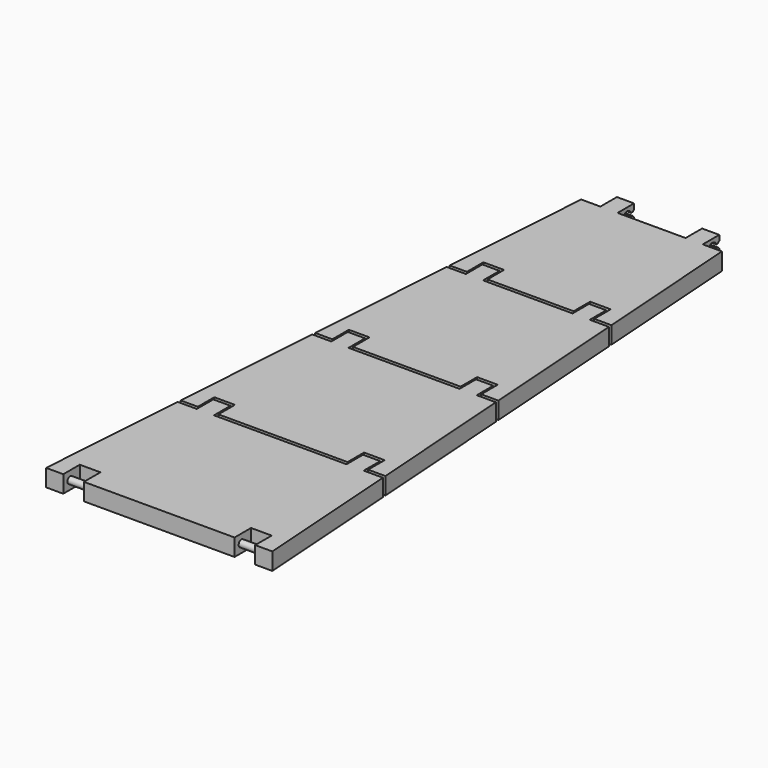
from build123d import *

# Parameters (mm, degrees)
F1_DEPTH  = 5
F12_START = -5.7
F10_R     = 1
F12_DEPTH = 62
F13_START = -5.5
F9_R      = 1.5
F9_R_2    = 1
F13_DEPTH = 55.3
F14_START = -6
F14_DEPTH = 56.6
F15_START = -6.3
F8_R      = 1.5
F8_R_2    = 1
F15_DEPTH = 49.5
F16_START = -5.7
F16_DEPTH = 49
F17_START = -6
F7_R      = 1.5
F7_R_2    = 1
F17_DEPTH = 43.6
F18_START = -5.7
F18_DEPTH = 42.3
F19_DEPTH = 45.5
F20_SIZE  = 0.5


with BuildPart() as f1:
    # F0 (on Top) → F1 (new body)
    with BuildSketch(Plane.XY):
        Polygon((-20.4571957112, 87.1), (-23.5168766766, 43.1), (-18.5168766766, 43.1), (-18.5168766766, 49.1), (-12.5168766766, 49.1), (-12.5168766766, 43.1), (12.5168766766, 43.1), (12.5168766766, 49.1), (18.5168766766, 49.1), (18.5168766766, 43.1), (23.5168766766, 43.1), (20.4571957112, 87.1), (14.8876575074, 87.1), (14.8876575074, 93.1), (9.8876575074, 93.1), (9.8876575074, 87.1), (-9.8876575074, 87.1), (-9.8876575074, 93.1), (-14.8876575074, 93.1), (-14.8876575074, 87.1), align=None)
    extrude(amount=F1_DEPTH)



with BuildPart() as f1b:
    # F0 (on Top) → F1, piece 2 (new body)
    with BuildSketch(Plane.XY):
        Polygon((-23.5864148803, 42.1), (-26.6460958457, -1.9), (-21.6460958457, -1.9), (-21.6460958457, 4.1), (-15.6460958457, 4.1), (-15.6460958457, -1.9), (15.6460958457, -1.9), (15.6460958457, 4.1), (21.6460958457, 4.1), (21.6460958457, -1.9), (26.6460958457, -1.9), (23.5864148803, 42.1), (18.0168766766, 42.1), (18.0168766766, 48.1), (13.0168766766, 48.1), (13.0168766766, 42.1), (-13.0168766766, 42.1), (-13.0168766766, 48.1), (-18.0168766766, 48.1), (-18.0168766766, 42.1), align=None)
    extrude(amount=F1_DEPTH)



with BuildPart() as f1c:
    # F0 (on Top) → F1, piece 3 (new body)
    with BuildSketch(Plane.XY):
        Polygon((-26.7156340495, -2.9), (-29.7753150149, -46.9), (-24.7753150149, -46.9), (-24.7753150149, -40.9), (-18.7753150149, -40.9), (-18.7753150149, -46.9), (18.7753150149, -46.9), (18.7753150149, -40.9), (24.7753150149, -40.9), (24.7753150149, -46.9), (29.7753150149, -46.9), (26.7156340495, -2.9), (21.1460958457, -2.9), (21.1460958457, 3.1), (16.1460958457, 3.1), (16.1460958457, -2.9), (-16.1460958457, -2.9), (-16.1460958457, 3.1), (-21.1460958457, 3.1), (-21.1460958457, -2.9), align=None)
    extrude(amount=F1_DEPTH)



with BuildPart() as f1d:
    # F0 (on Top) → F1, piece 4 (new body)
    with BuildSketch(Plane.XY):
        Polygon((-29.8448532186, -47.9), (-32.904534184, -91.9), (-27.904534184, -91.9), (-27.904534184, -85.9), (-21.904534184, -85.9), (-21.904534184, -91.9), (21.904534184, -91.9), (21.904534184, -85.9), (27.904534184, -85.9), (27.904534184, -91.9), (32.904534184, -91.9), (29.8448532186, -47.9), (24.2753150149, -47.9), (24.2753150149, -41.9), (19.2753150149, -41.9), (19.2753150149, -47.9), (-19.2753150149, -47.9), (-19.2753150149, -41.9), (-24.2753150149, -41.9), (-24.2753150149, -47.9), align=None)
    extrude(amount=F1_DEPTH)

    # F10 (on offset) → F12 (join)
    with BuildSketch(Plane.YZ.offset(36.904534184).offset(F12_START)):
        with Locations((-89.4, 2.5)):
            Circle(F10_R)
    extrude(amount=-F12_DEPTH)

    # F9 (on offset) → F13 (cut)
    with BuildSketch(Plane.YZ.offset(34.2753150149).offset(F13_START)):
        with Locations((-44.4, 2.5)):
            Circle(F9_R)
        with Locations((-44.4, 2.5)):
            Circle(F9_R_2, mode=Mode.SUBTRACT)
    extrude(amount=-F13_DEPTH, mode=Mode.SUBTRACT)


with BuildPart() as f1c_1:
    add(f1c.part)

    add(f1d.part)  # F14 merges F1d
    # F9 (on offset) → F14 (join)
    with BuildSketch(Plane.YZ.offset(34.2753150149).offset(F14_START)):
        with Locations((-44.4, 2.5)):
            Circle(F9_R_2)
    extrude(amount=-F14_DEPTH)

    # F8 (on offset) → F15 (cut)
    with BuildSketch(Plane.YZ.offset(31.1460958457).offset(F15_START)):
        with Locations((0.6, 2.5)):
            Circle(F8_R)
        with Locations((0.6, 2.5)):
            Circle(F8_R_2, mode=Mode.SUBTRACT)
    extrude(amount=-F15_DEPTH, mode=Mode.SUBTRACT)


with BuildPart() as f1b_1:
    add(f1b.part)

    add(f1c_1.part)  # F16 merges F1c
    # F8 (on offset) → F16 (join)
    with BuildSketch(Plane.YZ.offset(31.1460958457).offset(F16_START)):
        with Locations((0.6, 2.5)):
            Circle(F8_R_2)
    extrude(amount=-F16_DEPTH)

    # F7 (on offset) → F17 (cut)
    with BuildSketch(Plane.YZ.offset(28.0168766766).offset(F17_START)):
        with Locations((45.6, 2.5)):
            Circle(F7_R)
        with Locations((45.6, 2.5)):
            Circle(F7_R_2, mode=Mode.SUBTRACT)
    extrude(amount=-F17_DEPTH, mode=Mode.SUBTRACT)


with BuildPart() as f1_1:
    add(f1.part)

    add(f1b_1.part)  # F18 merges F1b
    # F7 (on offset) → F18 (join)
    with BuildSketch(Plane.YZ.offset(28.0168766766).offset(F18_START)):
        with Locations((45.6, 2.5)):
            Circle(F7_R_2)
    extrude(amount=-F18_DEPTH)

    # F11 (on offset) → F19 (cut)
    with BuildSketch(Plane.YZ.offset(24.8876575074)):
        with BuildLine():
            Line((95.6, 3), (92.0142135624, 3))
            ThreePointArc((92.0142135624, 3), (90.4708684127, 3.9944313411), (89.1209800542, 2.75))
            Line((89.1209800542, 2.75), (88.1, 2.75))
            Line((88.1, 2.75), (88.1, 2.25))
            Line((88.1, 2.25), (89.1209800542, 2.25))
            ThreePointArc((89.1209800542, 2.25), (90.4708684127, 1.0055686589), (92.0142135624, 2))
            Line((92.0142135624, 2), (95.6, 2))
            Line((95.6, 2), (95.6, 3))
        make_face()
    extrude(amount=-F19_DEPTH, mode=Mode.SUBTRACT)

    # F20
    f20_edges = [f1_1.edges().sort_by_distance(p)[0] for p in [
        (-12.387658, 93.1, 3),
        (-12.387658, 93.1, 2),
        (12.387658, 93.1, 3),
        (12.387658, 93.1, 2),
    ]]
    chamfer(f20_edges, length=F20_SIZE)


solid = f1_1.part
